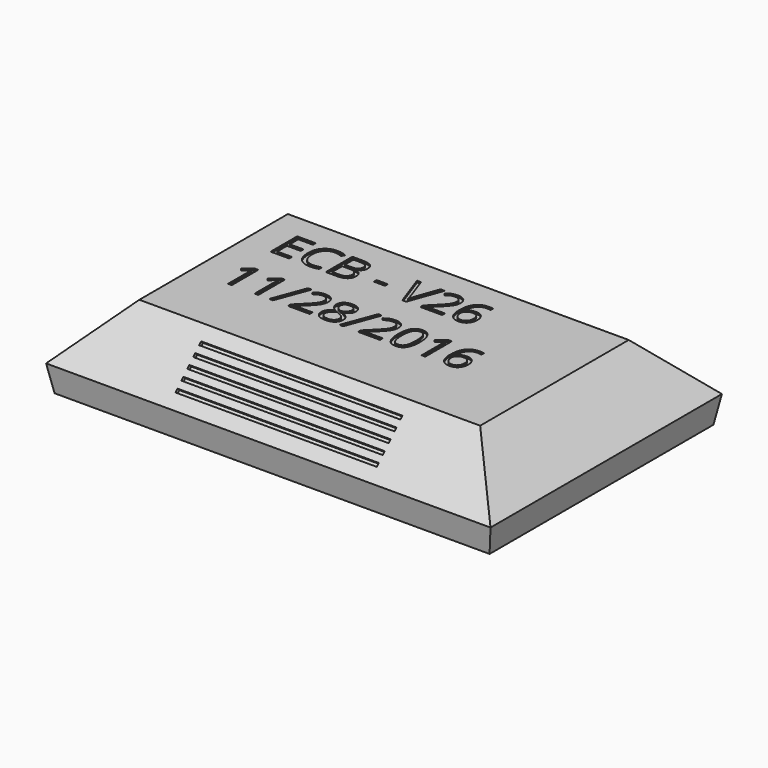
from build123d import *

# Parameters (mm, degrees)
F1_DEPTH      = 25
F2_SIZE       = 15
F3_T          = -1.5
F4_T1_DEPTH   = 184.9178535213
F4_T3_DEPTH   = 140.4178535213
F7_W          = 9.6
F7_H          = 19.5
F7_W_2        = 3.6
F7_H_2        = 5
F7_H_3        = 4.3857726092
F8_DEPTH      = 15
F10_W         = 9.6
F10_H         = 19.5
F11_DEPTH     = 8.75
F13_W         = 5
F13_H         = 6.5
F13_W_2       = 3.6
F13_H_2       = 6
F13_W_3       = 79.3071517747
F14_DEPTH     = 5.5
F15_W         = 57.75
F15_H         = 1
F16_DEPTH     = 1
F17_W         = 57.75
F17_H         = 1
F18_DEPTH     = 0.5
F19_TEXT_SIZE = 13.3258445809
F20_DEPTH     = 0.5


# Not quite as in the source:
# - a fillet or chamfer that OpenCascade refuses, or shapes differently, is made with other operations: its cross-section is extruded or revolved along the edge and cut away or added
# - Text() gives the source's letters only with a copy of the font that has no kerning and outlines rounded to 1/6400 em; it was checked with that copy


with BuildPart() as f1:
    # F0 (on Top) → F1 (new body)
    with BuildSketch(Plane.XY):
        Polygon((0, 1.5), (0, 0), (1.5, 0), (127.75, 0), (127.75, 81.75), (127.75, 83.25), (126.25, 83.25), (0, 83.25), align=None)
    extrude(amount=F1_DEPTH)

    # F2
    f2_edges = [f1.edges().sort_by_distance(p)[0] for p in [
        (63.875, 0, 25),
        (63.875, 83.25, 25),
        (127.75, 41.625, 25),
        (0, 41.625, 25),
    ]]
    chamfer(f2_edges, length=F2_SIZE)

    # F3
    f3_openings = [f1.faces().sort_by_distance(p)[0] for p in [
        (63.875, 41.625, 0),
    ]]
    offset(amount=F3_T, openings=f3_openings)

    # F4: chamfer of 11 x 1.9395967878 on 4 edges, made by hand

    # F4_s2 → F4_t1 (cut)
    with BuildSketch(Plane.YZ.offset(-28.5839267606)):
        Polygon((0, 11), (1.9395967878, 0), (0, 0), align=None)
        Polygon((83.25, 11), (81.3104032122, 0), (83.25, 0), align=None)
    extrude(amount=F4_T1_DEPTH, mode=Mode.SUBTRACT)

    # F4_s4 → F4_t3 (cut)
    with BuildSketch(Plane.XZ.offset(-111.8339267606)):
        Polygon((0, 11), (1.9395967878, 0), (0, 0), align=None)
        Polygon((127.75, 11), (125.8104032122, 0), (127.75, 0), align=None)
    extrude(amount=F4_T3_DEPTH, mode=Mode.SUBTRACT)

    # F7 (on face) → F8 (join)
    with BuildSketch(Plane.XY.offset(25)):
        Polygon((20.6213203436, 58.1213203436), (15.6213203436, 58.1213203436), (15.6213203436, 26.6213203436), (20.6213203436, 26.6213203436), (24.2213203436, 26.6213203436), (29.2213203436, 26.6213203436), (29.2213203436, 58.1213203436), (24.2213203436, 58.1213203436), align=None)
        with Locations((22.4213203436, 42.3713203436)):
            Rectangle(F7_W, F7_H, mode=Mode.SUBTRACT)
        with Locations((22.4213203436, 60.6213203436)):
            Rectangle(F7_W_2, F7_H_2)
        with Locations((22.4213203436, 24.1213203436)):
            Rectangle(F7_W_2, F7_H_2)
        Polygon((103.5284721182, 58.1213203436), (98.5284721182, 58.1213203436), (98.5284721182, 26.6213203436), (103.5284721182, 26.6213203436), (107.1284721182, 26.6213203436), (112.1284721182, 26.6213203436), (112.1284721182, 58.1213203436), (107.1284721182, 58.1213203436), align=None)
        with Locations((105.3284721182, 42.3713203436)):
            Rectangle(F7_W, F7_H, mode=Mode.SUBTRACT)
        with Locations((105.3284721182, 60.3142066481)):
            Rectangle(F7_W_2, F7_H_3)
        with Locations((105.3284721182, 24.1213203436)):
            Rectangle(F7_W_2, F7_H_2)
    extrude(amount=-F8_DEPTH)

    # F10 (on offset) → F11 (join)
    with BuildSketch(Plane(origin=(0, 0, 23.5), x_dir=(1, 0, 0), z_dir=(0, 0, -1))):
        with Locations((22.4213203436, -42.3713203436)):
            Rectangle(F10_W, F10_H)
        with Locations((105.3284721182, -42.3713203436)):
            Rectangle(F10_W, F10_H)
    extrude(amount=F11_DEPTH)

    # F13 (on offset) → F14 (cut)
    with BuildSketch(Plane(origin=(0, 0, 10), x_dir=(1, 0, 0), z_dir=(0, 0, -1))):
        with Locations((18.1213203436, -42.3713203436)):
            Rectangle(F13_W, F13_H)
        with Locations((22.4213203436, -42.3713203436)):
            Rectangle(F13_W_2, F13_H)
        with Locations((22.4213203436, -48.6213203436)):
            Rectangle(F13_W_2, F13_H_2)
        with Locations((63.8748962309, -42.3713203436)):
            Rectangle(F13_W_3, F13_H)
        with Locations((22.4213203436, -36.1213203436)):
            Rectangle(F13_W_2, F13_H_2)
        with Locations((105.3284721182, -42.3713203436)):
            Rectangle(F13_W_2, F13_H)
        with Locations((105.3284721182, -48.6213203436)):
            Rectangle(F13_W_2, F13_H_2)
        with Locations((109.6284721182, -42.3713203436)):
            Rectangle(F13_W, F13_H)
        with Locations((105.3284721182, -36.1213203436)):
            Rectangle(F13_W_2, F13_H_2)
    extrude(amount=-F14_DEPTH, mode=Mode.SUBTRACT)

    # F15 (on face) → F16 (cut)
    with BuildSketch(Plane(origin=(0, -5, 5), x_dir=(1, 0, 0), z_dir=(0, -0.7071067812, 0.7071067812))):
        with Locations((63.875, 20.7842712475)):
            Rectangle(F15_W, F15_H)
        with Locations((63.875, 17.7842712475)):
            Rectangle(F15_W, F15_H)
        with Locations((63.875, 14.7842712475)):
            Rectangle(F15_W, F15_H)
        with Locations((63.875, 23.7842712475)):
            Rectangle(F15_W, F15_H)
        with Locations((63.875, 11.7842712475)):
            Rectangle(F15_W, F15_H)
    extrude(amount=-F16_DEPTH, mode=Mode.SUBTRACT)

    # F17 (on face) → F18 (cut)
    with BuildSketch(Plane(origin=(0, 46.625, 46.625), x_dir=(-1, 0, 0), z_dir=(0, 0.7071067812, 0.7071067812))):
        with Locations((-63.875, -35.0823682863)):
            Rectangle(F17_W, F17_H)
        with Locations((-63.875, -38.0823682863)):
            Rectangle(F17_W, F17_H)
        with Locations((-63.875, -41.0823682863)):
            Rectangle(F17_W, F17_H)
        with Locations((-63.875, -44.0823682863)):
            Rectangle(F17_W, F17_H)
        with Locations((-63.875, -47.0823682863)):
            Rectangle(F17_W, F17_H)
    extrude(amount=-F18_DEPTH, mode=Mode.SUBTRACT)

    # F19 (on face) → F20 (cut)
    with BuildSketch(Plane.XY.offset(25)):
        with Locations((22.0851544291, 51.5927299857)):
            Text('ECB - V26', F19_TEXT_SIZE, font='Open Sans', text_align=(TextAlign.LEFT, TextAlign.BOTTOM))
        with Locations((22.0851544291, 33.4695813557)):
            Text('11/28/2016', F19_TEXT_SIZE, font='Open Sans', text_align=(TextAlign.LEFT, TextAlign.BOTTOM))
    extrude(amount=-F20_DEPTH, mode=Mode.SUBTRACT)


solid = f1.part
